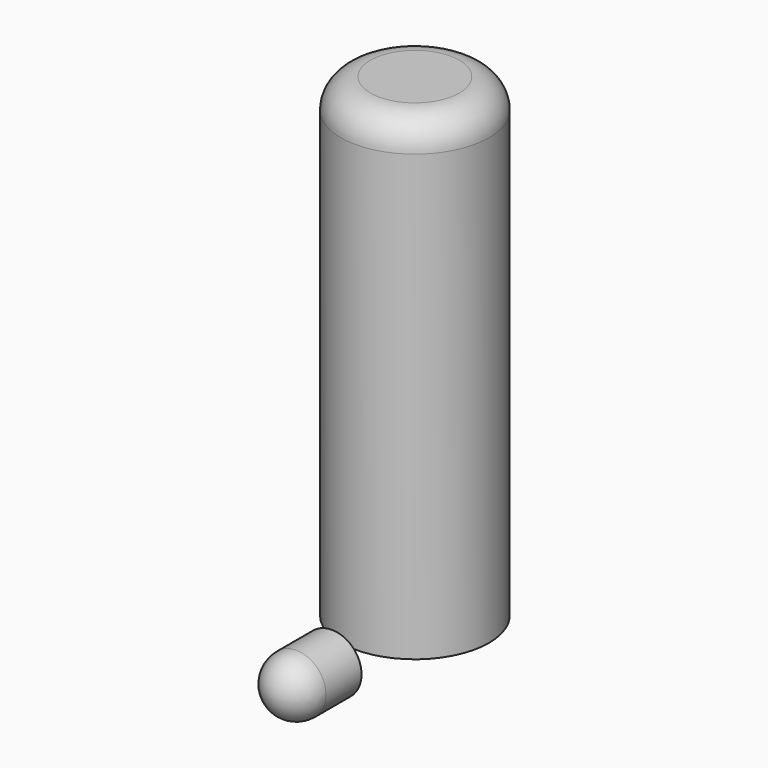
from build123d import *

# Parameters (mm, degrees)
F0_R      = 12.7
F1_DEPTH  = 76.2
F2_DEPTH  = 5.08
F3_R      = 5.08
F9_R      = 5.08
F10_DEPTH = 12.7
F11_R     = 5.08


with BuildPart() as f1:
    # F0 (on Top) → F1 (new body)
    with BuildSketch(Plane.XY):
        Circle(F0_R)
    extrude(amount=F1_DEPTH)

    # F2 (add): a face of the model
    f2_faces = [f1.faces().sort_by_distance(p)[0] for p in [
        (0, 0, 76.2),
    ]]
    extrude(f2_faces, amount=F2_DEPTH)

    # F3
    f3_edges = [f1.edges().sort_by_distance(p)[0] for p in [
        (-12.7, 0, 81.28),
    ]]
    fillet(f3_edges, radius=F3_R)


with BuildPart() as f10:
    # F9 (on plane+point) → F10 (new body)
    with BuildSketch(Plane.XZ.offset(17.78)):
        Circle(F9_R)
    extrude(amount=F10_DEPTH)

    # F11
    f11_edges = [f10.edges().sort_by_distance(p)[0] for p in [
        (-5.08, -30.48, 0),
    ]]
    fillet(f11_edges, radius=F11_R)


solid = Compound([f1.part, f10.part])
